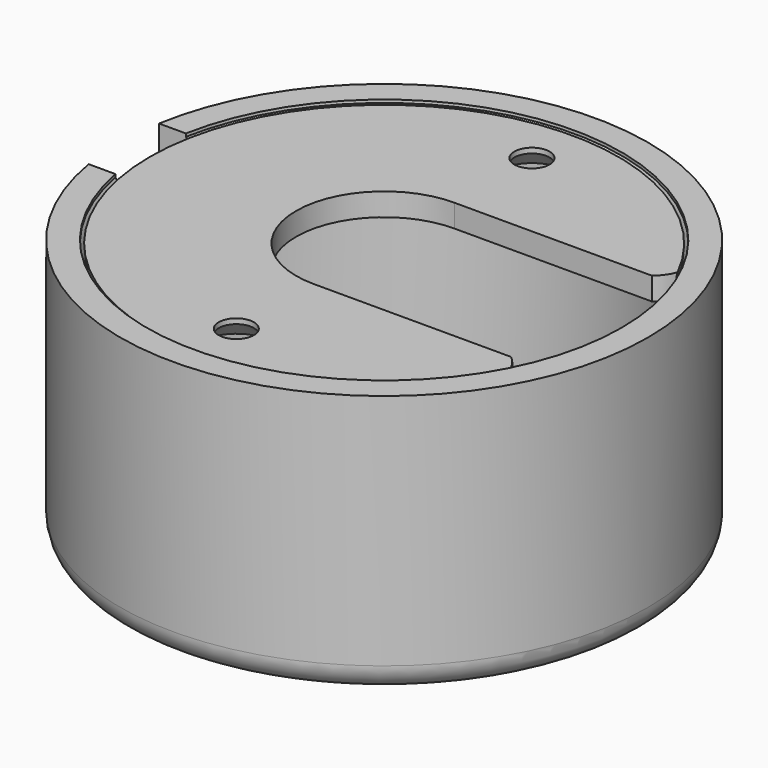
from build123d import *

# Parameters (mm, degrees)
F7_DEPTH        = 25
F9_DEPTH        = 25
F11_D           = 4
F11_CSINK_D     = 8
F11_CSINK_ANGLE = 90
F13_DEPTH       = 30.001


# Not quite as in the source:
# - a feature of the source that left no trace in its solid (it failed there, or was rolled back) is left out


with BuildPart() as f1:
    # F0 (on Front) → F1 (revolve)
    with BuildSketch(Plane.XZ):
        with BuildLine():
            Line((0, 3), (0, 0))
            Line((0, 0), (27, 0))
            ThreePointArc((27, 0), (29.1213203436, 0.8786796564), (30, 3))
            Line((30, 3), (30, 30))
            Line((30, 30), (27, 30))
            Line((27, 30), (27, 29.659981063))
            ThreePointArc((27, 29.659981063), (26.5313694768, 28.3675268292), (27, 27.0750725955))
            Line((27, 27.0750725955), (27, 3))
            Line((27, 3), (0, 3))
        make_face()
    revolve(axis=Axis((0, 0, 20.7135844976), (0, 0, 1)))

    # F12 (on Right) → F13 (cut, through all)
    with BuildSketch(Plane.YZ):
        with BuildLine():
            Line((5, 24.3423475833), (5, 32.1951069077))
            Line((5, 32.1951069077), (-5, 32.5018552183))
            Line((-5, 32.5018552183), (-5, 24.3423475833))
            ThreePointArc((-5, 24.3423475833), (0, 19.3423475833), (5, 24.3423475833))
        make_face()
    extrude(amount=-F13_DEPTH, mode=Mode.SUBTRACT)


with BuildPart() as f2:
    # F0 (on Front) → F2 (revolve)
    with BuildSketch(Plane.XZ):
        with BuildLine():
            Line((0, 27.0750725955), (27, 27.0750725955))
            ThreePointArc((27, 27.0750725955), (26.5313694768, 28.3675268292), (27, 29.659981063))
            Line((27, 29.659981063), (0, 29.659981063))
            Line((0, 29.659981063), (0, 27.0750725955))
        make_face()
    revolve(axis=Axis((0, 0, 20.7135844976), (0, 0, 1)))

    # F4 (on Front) → F5 (revolve, cut)
    with BuildSketch(Plane.XZ):
        with BuildLine():
            Line((27.2429585457, 29.4521301985), (27.0748790354, 30.6622516364))
            ThreePointArc((27.0748790354, 30.6622516364), (26.5911281972, 29.5003878586), (26.570642367, 28.2420068979))
            Line((26.570642367, 28.2420068979), (27.2429585457, 29.4521301985))
        make_face()
    revolve(axis=Axis((0, 0, 20.7135844976), (0, 0, 1)), mode=Mode.SUBTRACT)

    # F6 (on face) → F7 (cut)
    with BuildSketch(Plane.XY.offset(29.659981063)):
        with BuildLine():
            ThreePointArc((0, -10), (7.0710678119, -7.0710678119), (10, 0))
            ThreePointArc((10, 0), (7.0710678119, 7.0710678119), (0, 10))
            ThreePointArc((0, 10), (-10, 0), (0, -10))
        make_face()
        with BuildLine():
            ThreePointArc((0, 10), (7.0710678119, 7.0710678119), (10, 0))
            ThreePointArc((10, 0), (7.0710678119, -7.0710678119), (0, -10))
            Line((0, -10), (44.3025864661, -10))
            Line((44.3025864661, -10), (43.6370521784, 10))
            Line((43.6370521784, 10), (0, 10))
        make_face()
    extrude(amount=-F7_DEPTH, mode=Mode.SUBTRACT)

    # F8 (on face) → F9 (cut)
    with BuildSketch(Plane.XY.offset(29.659981063)):
        with BuildLine():
            ThreePointArc((23.9879842848, 14.1842635348), (22.7204724664, 10.2545780002), (18.7441203743, 9.1420859098))
            Line((18.7441203743, 9.1420859098), (19.8477320373, 7.0414338261))
            Line((19.8477320373, 7.0414338261), (30.4011907429, 7.6118907891))
            Line((30.4011907429, 7.6118907891), (23.9879842848, 14.1842635348))
        make_face()
        with BuildLine():
            Line((19.8477320373, -7.0414338261), (18.7441203743, -9.1420859098))
            ThreePointArc((18.7441203743, -9.1420859098), (22.7204724664, -10.2545780002), (23.9879842848, -14.1842635348))
            Line((23.9879842848, -14.1842635348), (30.4011907429, -7.6118907891))
            Line((30.4011907429, -7.6118907891), (19.8477320373, -7.0414338261))
        make_face()
    extrude(amount=-F9_DEPTH, mode=Mode.SUBTRACT)

    # F11 (through all)
    with Locations(Plane(origin=(0, 0, 27.0750725955), x_dir=(1, 0, 0), z_dir=(0, 0, -1))):
        with Locations((0, 21), (0, -21)):
            CounterSinkHole(F11_D / 2, F11_CSINK_D / 2, counter_sink_angle=F11_CSINK_ANGLE)


solid = Compound([f1.part, f2.part])
